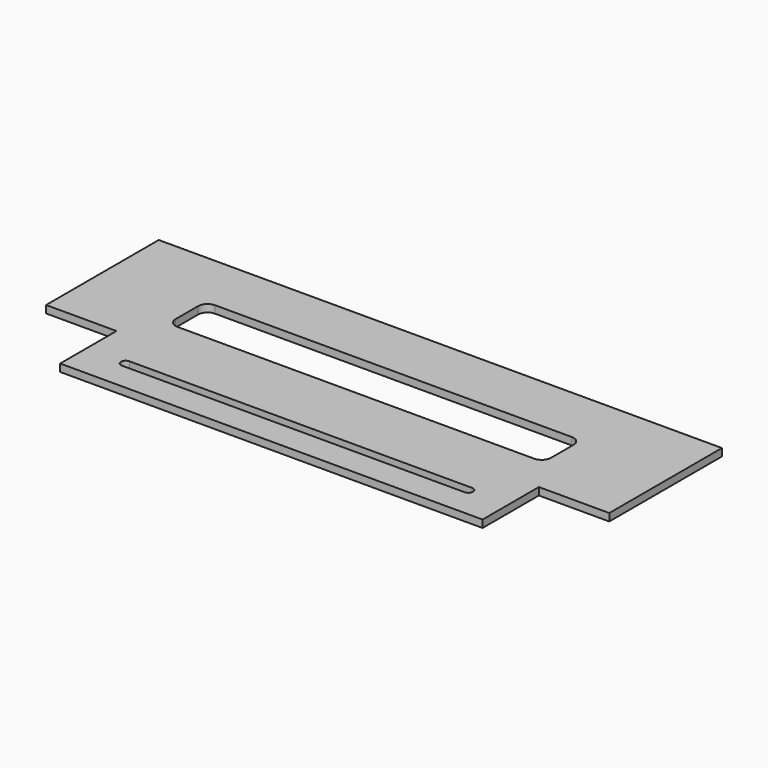
from build123d import *

# Parameters (mm, degrees)
F0_W     = 75
F0_H     = 2
F0_W_2   = 80
F0_H_2   = 10
F1_DEPTH = 1.59
F2_R     = 2
F3_R     = 0.99999


# Not quite as in the source:
# - a fillet or chamfer is up to 0.001 mm smaller than in the source, because OpenCascade refuses the exact size


with BuildPart() as f1:
    # F0 (on Top) → F1 (new body)
    with BuildSketch(Plane.XY):
        Polygon((45, 0), (-45, 0), (-60, 0), (-60, -30), (-45, -30), (-45, -45), (45, -45), (45, -30), (60, -30), (60, 0), align=None)
        with Locations((0, -38.175)):
            Rectangle(F0_W, F0_H, mode=Mode.SUBTRACT)
        with Locations((0, -17.5)):
            Rectangle(F0_W_2, F0_H_2, mode=Mode.SUBTRACT)
    extrude(amount=F1_DEPTH)

    # F2
    f2_edges = [f1.edges().sort_by_distance(p)[0] for p in [
        (40, -22.5, 0.795),
        (-40, -12.5, 0.795),
        (40, -12.5, 0.795),
        (-40, -22.5, 0.795),
    ]]
    fillet(f2_edges, radius=F2_R)

    # F3 (radius 1 in the source; OpenCascade refuses exactly that, so slightly less here)
    f3_edges = [f1.edges().sort_by_distance(p)[0] for p in [
        (-37.5, -37.175, 0.795),
        (37.5, -37.175, 0.795),
        (37.5, -39.175, 0.795),
        (-37.5, -39.175, 0.795),
    ]]
    fillet(f3_edges, radius=F3_R)


solid = f1.part
